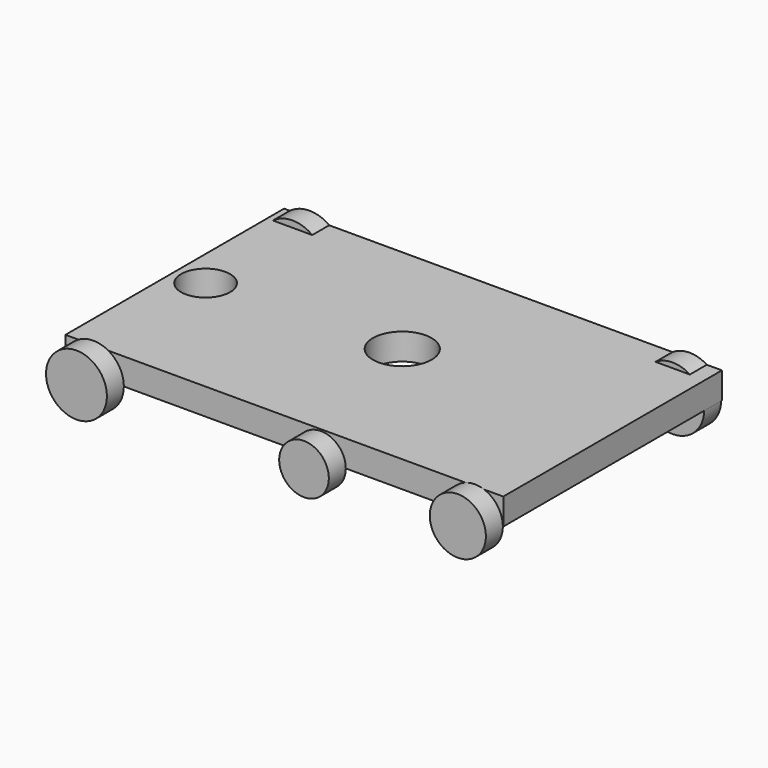
from build123d import *

# Parameters (mm, degrees)
F0_W      = 61.2648054957
F0_H      = 65.5319988728
F0_R      = 5.8807460694
F0_R_2    = 7.0457105262
F0_W_2    = 43.7088496983
F7_DEPTH  = 6.35
F8_R      = 7.297717767
F8_R_2    = 5.9512460605
F8_R_3    = 6.7280755045
F9_DEPTH  = 5.08
F10_R     = 5.1208570319
F10_R_2   = 7.9086669274
F10_R_3   = 7.5664721407
F11_DEPTH = 5.08
F12_R     = 3.7448458768
F12_R_2   = 3.5436310621
F12_R_3   = 3.2607470267
F12_R_4   = 3.6955687224
F13_DEPTH = 6.35


# Not quite as in the source:
# - the program builds the solid bodies; features that only make, move or delete a surface that nothing else refers to are left out


with BuildPart() as f7:
    # F0 (on Top) → F7 (new body)
    with BuildSketch(Plane.XY):
        with Locations((-30.6324027479, 0)):
            Rectangle(F0_W, F0_H)
        with Locations((-53.8736470044, 0)):
            Circle(F0_R, mode=Mode.SUBTRACT)
        with Locations((-8.4598210334, 2.1660252272)):
            Circle(F0_R_2, mode=Mode.SUBTRACT)
        with Locations((21.8544248492, 0)):
            Rectangle(F0_W_2, F0_H)
    extrude(amount=F7_DEPTH)

    # F8 (on face) → F9 (join)
    with BuildSketch(Plane.XZ.offset(32.7659994364)):
        with Locations((-54.5594133437, 0)):
            Circle(F8_R)
        Circle(F8_R_2)
        with Locations((36.8805900216, 0)):
            Circle(F8_R_3)
    extrude(amount=F9_DEPTH)

    # F10 (on face) → F11 (join)
    with BuildSketch(Plane.XZ.offset(-32.7659994364)):
        Circle(F10_R)
        with Locations((-55.1685914397, 0)):
            Circle(F10_R_2)
        with Locations((35.9666123986, 0)):
            Circle(F10_R_3)
    extrude(amount=F11_DEPTH)

    # F12 (on face) → F13 (join)
    with BuildSketch(Plane(origin=(0, 0, 0), x_dir=(1, 0, 0), z_dir=(0, 0, -1))):
        with Locations((30.5552948266, 4.8163635656)):
            Circle(F12_R)
        with Locations((30.5552948266, -3.6607212387)):
            Circle(F12_R_2)
        with Locations((21.4727055281, -3.6607212387)):
            Circle(F12_R_3)
        with Locations((21.4727055281, 4.8163635656)):
            Circle(F12_R_4)
    extrude(amount=F13_DEPTH)


solid = f7.part
